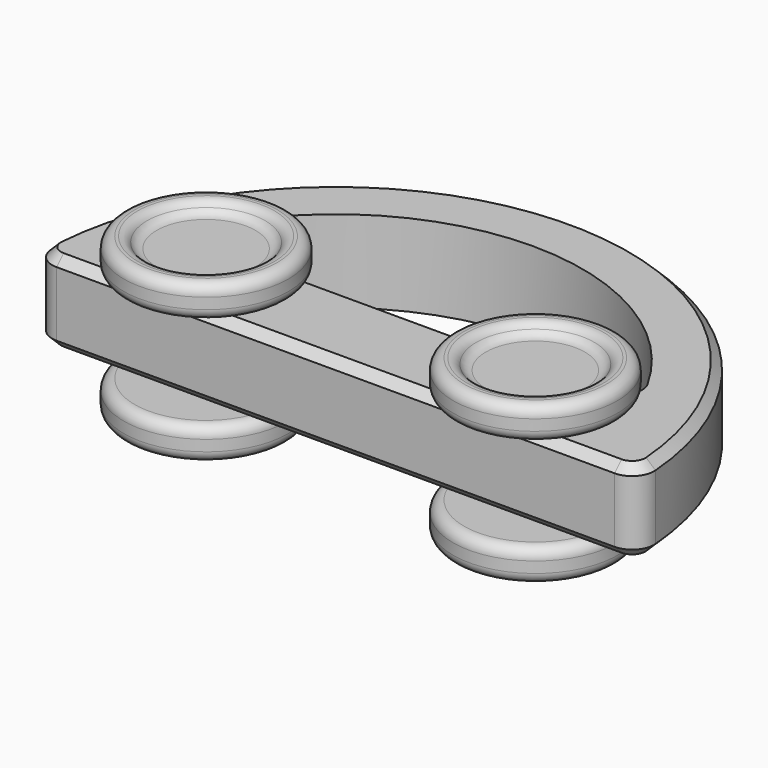
from build123d import *

# Parameters (mm, degrees)
F0_R     = 3.175
F1_DEPTH = 4.7625
F2_R     = 2.54
F4_R     = 9.525
F5_DEPTH = 3.81
F6_R     = 2.54
F7_DEPTH = 9.144
F8_R     = 6.6480864276
F9_DEPTH = 1.27
F10_R    = 1.26999
F11_R    = 1.27
F14_R    = 2.54
F15_SIZE = 1.016


# Not quite as in the source:
# - a fillet or chamfer is up to 0.001 mm smaller than in the source, because OpenCascade refuses the exact size


with BuildPart() as f1:
    # F0 (on Top) → F1 (new body, symmetric)
    with BuildSketch(Plane.XY):
        with BuildLine():
            ThreePointArc((-27.1072467382, -5.08), (-28.5465059417, 0.7362064244), (-26.2280401979, 6.2610992579))
            ThreePointArc((-26.2280401979, 6.2610992579), (0, 23.495), (26.2280401979, 6.2610992579))
            ThreePointArc((26.2280401979, 6.2610992579), (27.9689813848, 3.3432612906), (28.575, 0))
            ThreePointArc((28.575, 0), (28.2007076279, -2.6438938915), (27.1072467382, -5.08))
            Line((27.1072467382, -5.08), (34.925, -5.08))
            ThreePointArc((34.925, -5.08), (0, 29.845), (-34.925, -5.08))
            Line((-34.925, -5.08), (-27.1072467382, -5.08))
        make_face()
        with BuildLine():
            ThreePointArc((-10.9927532618, -5.08), (-9.8992923721, -2.6438938915), (-9.525, 0))
            ThreePointArc((-9.525, 0), (-9.8992923721, 2.6438938915), (-10.9927532618, 5.08))
            Line((-10.9927532618, 5.08), (-26.7077708729, 5.08))
            ThreePointArc((-26.7077708729, 5.08), (-26.4744928619, 5.6732252234), (-26.2280401979, 6.2610992579))
            ThreePointArc((-26.2280401979, 6.2610992579), (-28.5465059417, 0.7362064244), (-27.1072467382, -5.08))
            Line((-27.1072467382, -5.08), (-10.9927532618, -5.08))
        make_face()
        with Locations((-19.05, 0)):
            Circle(F0_R, mode=Mode.SUBTRACT)
        with BuildLine():
            ThreePointArc((-10.9927532618, 5.08), (-9.8992923721, 2.6438938915), (-9.525, 0))
            ThreePointArc((-9.525, 0), (-9.8992923721, -2.6438938915), (-10.9927532618, -5.08))
            Line((-10.9927532618, -5.08), (10.9927532618, -5.08))
            ThreePointArc((10.9927532618, -5.08), (9.525, 0), (10.9927532618, 5.08))
            Line((10.9927532618, 5.08), (-10.9927532618, 5.08))
        make_face()
        with BuildLine():
            Line((26.7077708729, 5.08), (10.9927532618, 5.08))
            ThreePointArc((10.9927532618, 5.08), (9.525, 0), (10.9927532618, -5.08))
            Line((10.9927532618, -5.08), (27.1072467382, -5.08))
            ThreePointArc((27.1072467382, -5.08), (28.2007076279, -2.6438938915), (28.575, 0))
            ThreePointArc((28.575, 0), (27.9689813848, 3.3432612906), (26.2280401979, 6.2610992579))
            ThreePointArc((26.2280401979, 6.2610992579), (26.4744928619, 5.6732252234), (26.7077708729, 5.08))
        make_face()
        with Locations((19.05, 0)):
            Circle(F0_R, mode=Mode.SUBTRACT)
    extrude(amount=F1_DEPTH, both=True)

    # F2
    f2_edges = [f1.edges().sort_by_distance(p)[0] for p in [
        (-26.707771, 5.08, 0),
    ]]
    fillet(f2_edges, radius=F2_R)

    # F14
    f14_edges = [f1.edges().sort_by_distance(p)[0] for p in [
        (-34.925, -5.08, 0),
        (26.707771, 5.08, 0),
        (34.925, -5.08, 0),
    ]]
    fillet(f14_edges, radius=F14_R)

    # F15
    f15_edges = [f1.edges().sort_by_distance(p)[0] for p in [
        (0, 29.845, 4.7625),
        (0, 29.845, -4.7625),
        (34.150394, -4.26418, 4.7625),
        (-34.150394, -4.26418, 4.7625),
        (0, -5.08, 4.7625),
        (34.150394, -4.26418, -4.7625),
        (-34.150394, -4.26418, -4.7625),
        (0, -5.08, -4.7625),
    ]]
    chamfer(f15_edges, length=F15_SIZE)


with BuildPart() as f5:
    # F4 (on offset) → F5 (new body)
    with BuildSketch(Plane.XY.offset(5.334)):
        with Locations((-19.05, 0)):
            Circle(F4_R)
    extrude(amount=F5_DEPTH)

    # F6 (on Top) → F7 (join, through all)
    with BuildSketch(Plane.XY):
        with Locations((-19.05, 0)):
            Circle(F6_R)
    extrude(amount=F7_DEPTH)

    # F8 (on face) → F9 (cut)
    with BuildSketch(Plane.XY.offset(9.144)):
        with Locations((-19.05, 0)):
            Circle(F8_R)
    extrude(amount=-F9_DEPTH, mode=Mode.SUBTRACT)

    # F10 (radius 1.27 in the source; OpenCascade refuses exactly that, so slightly less here)
    f10_edges = [f5.edges().sort_by_distance(p)[0] for p in [
        (-28.575, 0, 9.144),
        (-25.698086, 0, 9.144),
        (-28.575, 0, 5.334),
    ]]
    fillet(f10_edges, radius=F10_R)

    # F11
    f11_edges = [f5.edges().sort_by_distance(p)[0] for p in [
        (-25.698086, 0, 7.874),
    ]]
    fillet(f11_edges, radius=F11_R)

    # F12: F5 across plane


with BuildPart() as f5_1:
    add(f5.part)
    add(f5.part.mirror(Plane.XY))


with BuildPart() as f13_1:
    # F13: instance of F5
    add(f5_1.part.mirror(Plane.YZ))


solid = Compound([f1.part, f5_1.part, f13_1.part])
